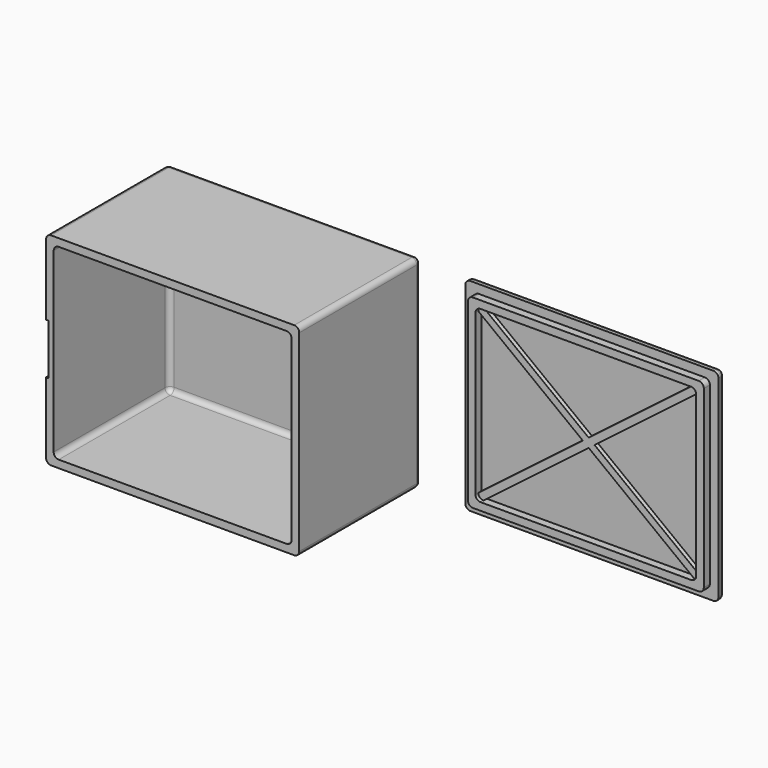
from build123d import *

# Parameters (mm, degrees)
F0_W         = 50
F0_H         = 40
F0_W_2       = 47
F0_H_2       = 37
F1_DEPTH     = 1.5
F0_W_3       = 46.6
F0_H_3       = 36.6
F0_W_4       = 43.6
F0_H_4       = 33.6
F2_DEPTH     = 30
F3_DEPTH     = 3
F4_R         = 1
F4_2_R       = 1
F6_DEPTH     = 0.8
F7_W         = 0.5
F7_H         = 10
F8_DEPTH     = 2
F9_T1_DEPTH  = 14.3301270189
F9_T6_DEPTH  = 3
F9_T11_DEPTH = 3


# Not quite as in the source:
# - a fillet or chamfer that OpenCascade refuses, or shapes differently, is made with other operations: its cross-section is extruded or revolved along the edge and cut away or added


with BuildPart() as f1:
    # F0 (on Front) → F1 (new body)
    with BuildSketch(Plane.XZ):
        with Locations((25, 20)):
            Rectangle(F0_W, F0_H)
        with Locations((25, 20)):
            Rectangle(F0_W_2, F0_H_2, mode=Mode.SUBTRACT)
        with Locations((25, 20)):
            Rectangle(F0_W_2, F0_H_2)
    extrude(amount=F1_DEPTH)

    # F0 (on Front) → F2 (join)
    with BuildSketch(Plane.XZ):
        with Locations((25, 20)):
            Rectangle(F0_W, F0_H)
        with Locations((25, 20)):
            Rectangle(F0_W_2, F0_H_2, mode=Mode.SUBTRACT)
    extrude(amount=F2_DEPTH)

    # F4
    f4_edges = [f1.edges().sort_by_distance(p)[0] for p in [
        (50, -15, 0),
        (0, -15, 0),
        (0, -15, 40),
        (50, -15, 40),
        (25, 0, 40),
        (0, 0, 20),
        (25, 0, 0),
        (50, 0, 20),
        (48.5, -15.75, 38.5),
        (48.5, -15.75, 1.5),
        (1.5, -15.75, 38.5),
        (1.5, -15.75, 1.5),
        (1.5, -1.5, 20),
        (25, -1.5, 38.5),
        (48.5, -1.5, 20),
        (25, -1.5, 1.5),
    ]]
    fillet(f4_edges, radius=F4_R)

    # F7 (on face) → F8 (cut)
    with BuildSketch(Plane.XZ.offset(30)):
        with Locations((0.25, 20)):
            Rectangle(F7_W, F7_H)
    extrude(amount=-F8_DEPTH, mode=Mode.SUBTRACT)

    # F9: fillet of radius 1 on 3 edges, made by hand

    # F9_s2 → F9_t1 (join)
    with BuildSketch(Plane.XY.offset(12.8349364905)):
        with BuildLine():
            ThreePointArc((0, -28), (0.3660254038, -28.3660254038), (0.5, -28.8660254038))
            Line((0.5, -28.8660254038), (0.5, -28))
            Line((0.5, -28), (0, -28))
        make_face()
    extrude(amount=F9_T1_DEPTH)


with BuildPart() as f1b:
    # F0 (on Front) → F1, piece 2 (new body)
    with BuildSketch(Plane.XZ):
        with Locations((85, 20)):
            Rectangle(F0_W, F0_H)
        with Locations((85, 20)):
            Rectangle(F0_W_3, F0_H_3, mode=Mode.SUBTRACT)
        with Locations((85, 20)):
            Rectangle(F0_W_3, F0_H_3)
        with Locations((85, 20)):
            Rectangle(F0_W_4, F0_H_4, mode=Mode.SUBTRACT)
        with Locations((85, 20)):
            Rectangle(F0_W_4, F0_H_4)
    extrude(amount=F1_DEPTH)

    # F0 (on Front) → F3 (join)
    with BuildSketch(Plane.XZ):
        with Locations((85, 20)):
            Rectangle(F0_W_3, F0_H_3)
        with Locations((85, 20)):
            Rectangle(F0_W_4, F0_H_4, mode=Mode.SUBTRACT)
    extrude(amount=F3_DEPTH)

    # F4#2
    f4_2_edges = [f1b.edges().sort_by_distance(p)[0] for p in [
        (85, 0, 40),
        (60, 0, 20),
        (85, 0, 0),
        (110, 0, 20),
        (60, -0.75, 0),
        (60, -0.75, 40),
        (110, -0.75, 40),
        (110, -0.75, 0),
        (61.7, -2.25, 1.7),
        (108.3, -2.25, 1.7),
        (108.3, -2.25, 38.3),
        (61.7, -2.25, 38.3),
        (63.2, -2.25, 36.8),
        (106.8, -2.25, 36.8),
        (106.8, -2.25, 3.2),
        (63.2, -2.25, 3.2),
    ]]
    fillet(f4_2_edges, radius=F4_2_R)

    # F5 (on face) → F6 (join)
    with BuildSketch(Plane.XZ.offset(1.5)):
        Polygon((85, 20.882629108), (83.8466257669, 20), (85, 19.117370892), (86.1533742331, 20), align=None)
        with BuildLine():
            Line((63.2, 35.8), (83.8466257669, 20))
            Line((83.8466257669, 20), (85, 20.882629108))
            Line((85, 20.882629108), (64.2, 36.8))
            ThreePointArc((64.2, 36.8), (63.4928932188, 36.5071067812), (63.2, 35.8))
        make_face()
        with BuildLine():
            Line((83.8466257669, 20), (63.2, 4.2))
            ThreePointArc((63.2, 4.2), (63.4928932188, 3.4928932188), (64.2, 3.2))
            Line((64.2, 3.2), (85, 19.117370892))
            Line((85, 19.117370892), (83.8466257669, 20))
        make_face()
        with BuildLine():
            Line((105.8, 36.8), (85, 20.882629108))
            Line((85, 20.882629108), (86.1533742331, 20))
            Line((86.1533742331, 20), (106.8, 35.8))
            ThreePointArc((106.8, 35.8), (106.5071067812, 36.5071067812), (105.8, 36.8))
        make_face()
        with BuildLine():
            Line((86.1533742331, 20), (85, 19.117370892))
            Line((85, 19.117370892), (105.8, 3.2))
            ThreePointArc((105.8, 3.2), (106.5071067812, 3.4928932188), (106.8, 4.2))
            Line((106.8, 4.2), (86.1533742331, 20))
        make_face()
    extrude(amount=F6_DEPTH)


with BuildPart() as f9_tool4:
    # F9_s5 → F9_t6 (new body)
    with BuildSketch(Plane.YZ):
        with BuildLine():
            ThreePointArc((-29, 15), (-28.2928932188, 15.2928932188), (-28, 16))
            Line((-28, 16), (-28, 15))
            Line((-28, 15), (-29, 15))
        make_face()
    extrude(amount=F9_T6_DEPTH)

    split(bisect_by=Plane.YZ.offset(1.5), keep=Keep.BOTTOM)


with BuildPart() as f1_1:
    add(f1.part)

    # F9_t3: union F9_tool4
    add(f9_tool4.part)


with BuildPart() as f9_tool9:
    # F9_s10 → F9_t11 (new body)
    with BuildSketch(Plane.YZ.offset(3)):
        with BuildLine():
            ThreePointArc((-28, 24), (-28.2928932188, 24.7071067812), (-29, 25))
            Line((-29, 25), (-28, 25))
            Line((-28, 25), (-28, 24))
        make_face()
    extrude(amount=-F9_T11_DEPTH)

    split(bisect_by=Plane.YZ.offset(1.5), keep=Keep.BOTTOM)


with BuildPart() as f1_2:
    add(f1_1.part)

    # F9_t8: union F9_tool9
    add(f9_tool9.part)


solid = Compound([f1b.part, f1_2.part])
